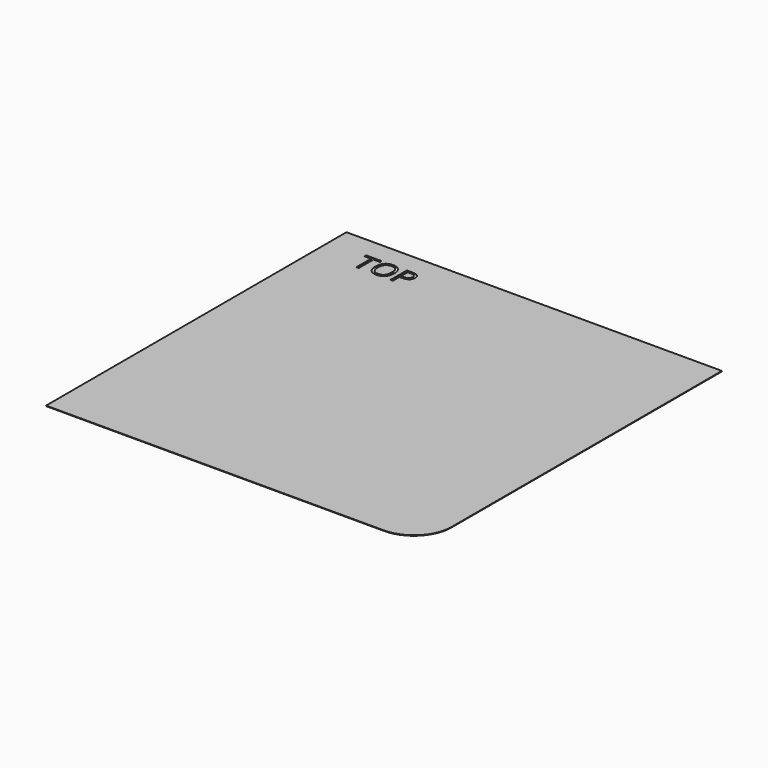
from build123d import *

# Parameters (mm, degrees)
F1_DEPTH     = 0.2
F2_TEXT_SIZE = 11.4447126786
F3_DEPTH     = 25


# Not quite as in the source:
# - Text() gives the source's letters only with a copy of the font that has no kerning and outlines rounded to 1/6400 em; it was checked with that copy


with BuildPart() as f1:
    # F0 (on Top) → F1 (new body)
    with BuildSketch(Plane.XY):
        with BuildLine():
            Line((0, 150), (0, 0))
            Line((0, 0), (135, 0))
            ThreePointArc((135, 0), (145.6066017178, 4.3933982822), (150, 15))
            Line((150, 15), (150, 150))
            Line((150, 150), (0, 150))
        make_face()
    extrude(amount=F1_DEPTH)

    # F2 (on face) → F3 (cut)
    with BuildSketch(Plane.XY):
        with Locations((14.4887007773, 133.4587037563)):
            Text('TOP', F2_TEXT_SIZE, font='Open Sans', text_align=(TextAlign.LEFT, TextAlign.BOTTOM))
    extrude(amount=F3_DEPTH, mode=Mode.SUBTRACT)


solid = f1.part
